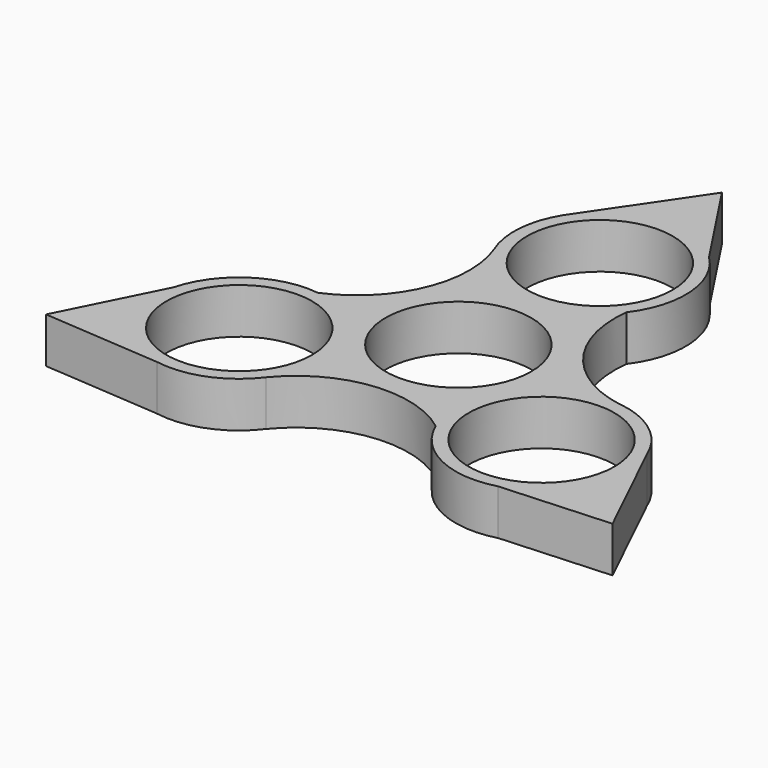
from build123d import *

# Parameters (mm, degrees)
F0_R     = 11.2
F1_DEPTH = 7


# Not quite as in the source:
# - ends of sketch curves that miss each other by under 0.0002 mm in the source are joined


with BuildPart() as f1:
    # F0 (on Top) → F1 (new body)
    with BuildSketch(Plane.XY):
        with BuildLine():
            ThreePointArc((24.885011592, 0), (13.8227560246, 6.7091569655), (10.5100821241, 19.2156543591))
            ThreePointArc((10.5100821241, 19.2156543591), (13.1664242497, 28.1426673783), (9.267685926, 36.601246125))
            Line((9.267685926, 36.601246125), (0, 50.6668537855))
            Line((0, 50.6668537855), (-10.6134602306, 35.0499921165))
            Line((-10.6134602306, 35.0499921165), (-11.2040059959, 34.1810510431))
            ThreePointArc((-11.2040059959, 34.1810510431), (-13.1594893438, 28.235141726), (-12.1560699163, 22.0568812763))
            ThreePointArc((-12.1560699163, 22.0568812763), (-12.4352425028, 9.122108449), (-21.6098500078, 0))
            ThreePointArc((-21.6098500078, 0), (-30.6478922927, -2.1487015261), (-36.0320947169, -9.7191574841))
            Line((-36.0320947169, -9.7191574841), (-43.5794253076, -24.7780127605))
            Line((-43.5794253076, -24.7780127605), (-25.4962357758, -26.1061598733))
            ThreePointArc((-25.4962357758, -26.1061598733), (-18.4080870059, -25.3666213531), (-12.7374420281, -21.0500769317))
            ThreePointArc((-12.7374420281, -21.0500769317), (-1.3959205219, -14.82446107), (11.0913608835, -18.2088500145))
            ThreePointArc((11.0913608835, -18.2088500145), (17.4993705689, -24.9467054642), (26.7596797789, -25.7881075822))
            ThreePointArc((26.7596797789, -25.7881075822), (35.0805283727, -18.9135515404), (35.4898237471, -8.127981579))
            ThreePointArc((35.4898237471, -8.127981579), (31.3336966338, -2.63072231), (24.9734656325, 0.0227120051))
            Line((24.9734656325, 0.0227120051), (24.885011592, 0))
        make_face()
        with Locations((-23.2474307999, -13.063953107)):
            Circle(F0_R, mode=Mode.SUBTRACT)
        with Locations((23.2474307999, -13.063953107)):
            Circle(F0_R, mode=Mode.SUBTRACT)
        Circle(F0_R, mode=Mode.SUBTRACT)
        with Locations((0, 27.2017781838)):
            Circle(F0_R, mode=Mode.SUBTRACT)
        with BuildLine():
            Line((43.5474583602, -24.7964688862), (35.4898237471, -8.127981579))
            ThreePointArc((35.4898237471, -8.127981579), (35.0805283727, -18.9135515404), (26.7596797789, -25.7881075822))
            Line((26.7596797789, -25.7881075822), (43.5474583602, -24.7964688862))
        make_face()
    extrude(amount=F1_DEPTH)


solid = f1.part
